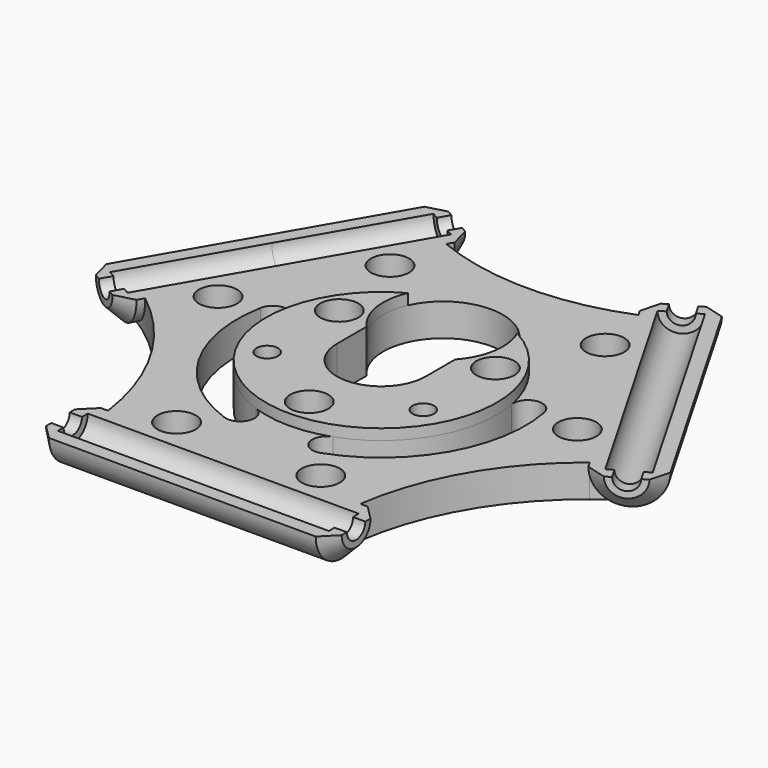
from build123d import *

# Parameters (mm, degrees)
F0_R            = 2.65
F0_R_2          = 1.5
F1_DEPTH        = 4.5
F2_R            = 1.6
F3_DEPTH        = 70.8788764306
F3_COPIES_COUNT = 3
F5_R            = 2.6
F6_DEPTH        = 18.8
F6_DEPTH_BACK   = 18.8
F6_COPIES_COUNT = 3
F8_T1_DEPTH     = 63.5
F8_T3_DEPTH     = 63.5
F8_T5_DEPTH     = 63.5
F8_T10_DEPTH    = 25.5
F8_S11_R        = 35.5
F8_T12_DEPTH    = 16
F8_T16_DEPTH    = 25.5
F8_S17_R        = 35.5
F8_T18_DEPTH    = 16
F8_T22_DEPTH    = 25.5
F8_S23_R        = 35.5
F8_T24_DEPTH    = 15
F8_T28_DEPTH    = 25.5
F8_S29_R        = 35.5
F8_T30_DEPTH    = 15
F8_T34_DEPTH    = 25.5
F8_S35_R        = 35.5
F8_T36_DEPTH    = 16
F8_T40_DEPTH    = 25.5
F8_S41_R        = 35.5
F8_T42_DEPTH    = 16
F9_SIZE         = 2
F10_R           = 1.5
F10_R_2         = 2.65
F11_DEPTH       = 1.5


# Not quite as in the source:
# - a fillet or chamfer that OpenCascade refuses, or shapes differently, is made with other operations: its cross-section is extruded or revolved along the edge and cut away or added
# - a pattern or mirror of a feature is missing from the dataset's text; its kind, count and spacing are read off the source's solid


with BuildPart() as f1:
    # F0 (on Top) → F1 (new body)
    with BuildSketch(Plane.XY):
        with BuildLine():
            Line((-40.1278764306, -0.5035207776), (-32.3336477965, -5.0035207776))
            Line((-32.3336477965, -5.0035207776), (-30.8336477965, -2.4054445662))
            ThreePointArc((-30.8336477965, -2.4054445662), (-21.9158664068, -12.6531313695), (-17.5, -25.5))
            Line((-17.5, -25.5), (-20.5, -25.5))
            Line((-20.5, -25.5), (-20.5, -34.5))
            Line((-20.5, -34.5), (20.5, -34.5))
            Line((20.5, -34.5), (20.5, -25.5))
            Line((20.5, -25.5), (17.5, -25.5))
            ThreePointArc((17.5, -25.5), (21.9158664068, -12.6531313695), (30.8336477965, -2.4054445662))
            Line((30.8336477965, -2.4054445662), (32.3336477965, -5.0035207776))
            Line((32.3336477965, -5.0035207776), (40.1278764306, -0.5035207776))
            Line((40.1278764306, -0.5035207776), (19.6278764306, 35.0035207776))
            Line((19.6278764306, 35.0035207776), (11.8336477965, 30.5035207776))
            Line((11.8336477965, 30.5035207776), (13.3336477965, 27.9054445662))
            ThreePointArc((13.3336477965, 27.9054445662), (0, 25.306262739), (-13.3336477965, 27.9054445662))
            Line((-13.3336477965, 27.9054445662), (-11.8336477965, 30.5035207776))
            Line((-11.8336477965, 30.5035207776), (-19.6278764306, 35.0035207776))
            Line((-19.6278764306, 35.0035207776), (-40.1278764306, -0.5035207776))
        make_face()
        with Locations((-10, -23)):
            Circle(F0_R, mode=Mode.SUBTRACT)
        with BuildLine():
            ThreePointArc((-19.6632649519, 3.6545877239), (-17.3314796843, 5.2554554467), (-15.7306119615, 2.9236701791))
            ThreePointArc((-15.7306119615, 2.9236701791), (-13.8564064606, -8), (-5.3333333333, -15.0849446653))
            ThreePointArc((-5.3333333333, -15.0849446653), (-4.1143819168, -17.6372294151), (-6.6666666667, -18.8561808316))
            ThreePointArc((-6.6666666667, -18.8561808316), (-17.3205080757, -10), (-19.6632649519, 3.6545877239))
        make_face(mode=Mode.SUBTRACT)
        with Locations((-10.8253175473, -6.25)):
            Circle(F0_R_2, mode=Mode.SUBTRACT)
        with Locations((10, -23)):
            Circle(F0_R, mode=Mode.SUBTRACT)
        with Locations((0, -12.5)):
            Circle(F0_R, mode=Mode.SUBTRACT)
        with BuildLine():
            ThreePointArc((5.3333333333, -15.0849446653), (13.8564064606, -8), (15.7306119615, 2.9236701791))
            ThreePointArc((15.7306119615, 2.9236701791), (17.3314796843, 5.2554554467), (19.6632649519, 3.6545877239))
            ThreePointArc((19.6632649519, 3.6545877239), (17.3205080757, -10), (6.6666666667, -18.8561808316))
            ThreePointArc((6.6666666667, -18.8561808316), (4.1143819168, -17.6372294151), (5.3333333333, -15.0849446653))
        make_face(mode=Mode.SUBTRACT)
        with Locations((10.8253175473, -6.25)):
            Circle(F0_R_2, mode=Mode.SUBTRACT)
        with Locations((-24.918584287, 2.8397459622)):
            Circle(F0_R, mode=Mode.SUBTRACT)
        with Locations((-10.8253175473, 6.25)):
            Circle(F0_R, mode=Mode.SUBTRACT)
        with BuildLine():
            ThreePointArc((6.15, 0), (0, -6.15), (-6.15, 0))
            Line((-6.15, 0), (-6.15, 5.1163952154))
            ThreePointArc((-6.15, 5.1163952154), (0, 18.990217961), (6.15, 5.1163952154))
            Line((6.15, 5.1163952154), (6.15, 0))
        make_face(mode=Mode.SUBTRACT)
        with Locations((-14.918584287, 20.1602540378)):
            Circle(F0_R, mode=Mode.SUBTRACT)
        with Locations((10.8253175473, 6.25)):
            Circle(F0_R, mode=Mode.SUBTRACT)
        with Locations((24.918584287, 2.8397459622)):
            Circle(F0_R, mode=Mode.SUBTRACT)
        with Locations((14.918584287, 20.1602540378)):
            Circle(F0_R, mode=Mode.SUBTRACT)
    extrude(amount=F1_DEPTH)

    # F2 (on face) → F3 (cut, through all)
    with BuildSketch(Plane(origin=(-10.25, -17.7535207776, 0), x_dir=(0.8660254038, -0.5, 0), z_dir=(-0.5, -0.8660254038, 0))):
        with Locations((-30, 4.5)):
            Circle(F2_R)
    f3 = extrude(amount=-F3_DEPTH, mode=Mode.SUBTRACT)

    # F3_copies: F3 ×3 about axis
    f3_copies_axis = Axis((0, 0, 0), (0, 0, 1))
    for i in range(1, F3_COPIES_COUNT):
        add(f3.rotate(f3_copies_axis, i * 360 / F3_COPIES_COUNT), mode=Mode.SUBTRACT)

    # F5 (on plane+point) → F6 (cut, two sides)
    with BuildSketch(Plane(origin=(0, 0, 0), x_dir=(0.8660254038, -0.5, 0), z_dir=(-0.5, -0.8660254038, 0))) as f6_sk:
        with Locations((-30, 4.5)):
            Circle(F5_R)
    f6 = extrude(amount=-F6_DEPTH, mode=Mode.SUBTRACT) + extrude(f6_sk.sketch, amount=F6_DEPTH_BACK, mode=Mode.SUBTRACT)

    # F6_copies: F6 ×3 about axis
    f6_copies_axis = Axis((0, 0, 0), (0, 0, 1))
    for i in range(1, F6_COPIES_COUNT):
        add(f6.rotate(f6_copies_axis, i * 360 / F6_COPIES_COUNT), mode=Mode.SUBTRACT)

    # F8: fillet of radius 4.5 on 9 edges, made by hand

    # F8_s2 → F8_t1 (cut)
    with BuildSketch(Plane(origin=(15.875, 27.4963065702, 0), x_dir=(0, 0, 1), z_dir=(-0.5, -0.8660254038, 0))):
        with BuildLine():
            ThreePointArc((4.5, 34.5), (1.3180194847, 33.1819805153), (0, 30))
            Line((0, 30), (0, 34.5))
            Line((0, 34.5), (4.5, 34.5))
        make_face()
    extrude(amount=F8_T1_DEPTH, mode=Mode.SUBTRACT)

    # F8_s4 → F8_t3 (cut)
    with BuildSketch(Plane.YZ.offset(-31.75)):
        with BuildLine():
            ThreePointArc((-30, 0), (-33.1819805153, 1.3180194847), (-34.5, 4.5))
            Line((-34.5, 4.5), (-34.5, 0))
            Line((-34.5, 0), (-30, 0))
        make_face()
    extrude(amount=F8_T3_DEPTH, mode=Mode.SUBTRACT)

    # F8_s6 → F8_t5 (cut)
    with BuildSketch(Plane(origin=(15.875, -27.4963065702, 0), x_dir=(0, 0, 1), z_dir=(-0.5, 0.8660254038, 0))):
        with BuildLine():
            ThreePointArc((0, 30), (1.3180194847, 33.1819805153), (4.5, 34.5))
            Line((4.5, 34.5), (0, 34.5))
            Line((0, 34.5), (0, 30))
        make_face()
    extrude(amount=F8_T5_DEPTH, mode=Mode.SUBTRACT)


with BuildPart() as f8_tool8:
    # F8_s9 → F8_t10 (new body)
    with BuildSketch(Plane(origin=(-15.875, -27.4963065702, 0), x_dir=(0, 0, 1), z_dir=(0.5, 0.8660254038, 0))):
        with BuildLine():
            ThreePointArc((0, -30), (1.3180194847, -26.8180194847), (4.5, -25.5))
            Line((4.5, -25.5), (0, -25.5))
            Line((0, -25.5), (0, -30))
        make_face()
    extrude(amount=F8_T10_DEPTH)

    # F8_s11 → F8_t12 (intersect, symmetric)
    with BuildSketch(Plane.XY.offset(2.3)):
        with Locations((-52.6597682412, -30.4031313695)):
            Circle(F8_S11_R)
    extrude(amount=F8_T12_DEPTH, both=True, mode=Mode.INTERSECT)


with BuildPart() as f1_1:
    add(f1.part)

    # F8_t7: cut F8_tool8
    add(f8_tool8.part, mode=Mode.SUBTRACT)


with BuildPart() as f8_tool14:
    # F8_s15 → F8_t16 (new body)
    with BuildSketch(Plane(origin=(3.125, 5.4126587737, 0), x_dir=(0, 0, 1), z_dir=(0.5, 0.8660254038, 0))):
        with BuildLine():
            ThreePointArc((0, -30), (1.3180194847, -26.8180194847), (4.5, -25.5))
            Line((4.5, -25.5), (0, -25.5))
            Line((0, -25.5), (0, -30))
        make_face()
    extrude(amount=F8_T16_DEPTH)

    # F8_s17 → F8_t18 (intersect, symmetric)
    with BuildSketch(Plane.XY.offset(2.2)):
        with Locations((0, 60.806262739)):
            Circle(F8_S17_R)
    extrude(amount=F8_T18_DEPTH, both=True, mode=Mode.INTERSECT)


with BuildPart() as f1_2:
    add(f1_1.part)

    # F8_t13: cut F8_tool14
    add(f8_tool14.part, mode=Mode.SUBTRACT)


with BuildPart() as f8_tool20:
    # F8_s21 → F8_t22 (new body)
    with BuildSketch(Plane.YZ.offset(-6.25)):
        with BuildLine():
            ThreePointArc((-30, 0), (-26.8180194847, 1.3180194847), (-25.5, 4.5))
            Line((-25.5, 4.5), (-25.5, 0))
            Line((-25.5, 0), (-30, 0))
        make_face()
    extrude(amount=-F8_T22_DEPTH)

    # F8_s23 → F8_t24 (intersect, symmetric)
    with BuildSketch(Plane.XY.offset(2.2)):
        with Locations((-52.6597682412, -30.4031313695)):
            Circle(F8_S23_R)
    extrude(amount=F8_T24_DEPTH, both=True, mode=Mode.INTERSECT)


with BuildPart() as f1_3:
    add(f1_2.part)

    # F8_t19: cut F8_tool20
    add(f8_tool20.part, mode=Mode.SUBTRACT)


with BuildPart() as f8_tool26:
    # F8_s27 → F8_t28 (new body)
    with BuildSketch(Plane.YZ.offset(31.75)):
        with BuildLine():
            ThreePointArc((-30, 0), (-26.8180194847, 1.3180194847), (-25.5, 4.5))
            Line((-25.5, 4.5), (-25.5, 0))
            Line((-25.5, 0), (-30, 0))
        make_face()
    extrude(amount=-F8_T28_DEPTH)

    # F8_s29 → F8_t30 (intersect, symmetric)
    with BuildSketch(Plane.XY.offset(2.2)):
        with Locations((52.6597682412, -30.4031313695)):
            Circle(F8_S29_R)
    extrude(amount=F8_T30_DEPTH, both=True, mode=Mode.INTERSECT)


with BuildPart() as f1_4:
    add(f1_3.part)

    # F8_t25: cut F8_tool26
    add(f8_tool26.part, mode=Mode.SUBTRACT)


with BuildPart() as f8_tool32:
    # F8_s33 → F8_t34 (new body)
    with BuildSketch(Plane(origin=(3.125, -5.4126587737, 0), x_dir=(0, 0, 1), z_dir=(0.5, -0.8660254038, 0))):
        with BuildLine():
            ThreePointArc((0, -30), (1.3180194847, -26.8180194847), (4.5, -25.5))
            Line((4.5, -25.5), (0, -25.5))
            Line((0, -25.5), (0, -30))
        make_face()
    extrude(amount=F8_T34_DEPTH)

    # F8_s35 → F8_t36 (intersect, symmetric)
    with BuildSketch(Plane.XY.offset(2.3)):
        with Locations((52.6597682412, -30.4031313695)):
            Circle(F8_S35_R)
    extrude(amount=F8_T36_DEPTH, both=True, mode=Mode.INTERSECT)


with BuildPart() as f1_5:
    add(f1_4.part)

    # F8_t31: cut F8_tool32
    add(f8_tool32.part, mode=Mode.SUBTRACT)


with BuildPart() as f8_tool38:
    # F8_s39 → F8_t40 (new body)
    with BuildSketch(Plane(origin=(-15.875, 27.4963065702, 0), x_dir=(0, 0, 1), z_dir=(0.5, -0.8660254038, 0))):
        with BuildLine():
            ThreePointArc((0, -30), (1.3180194847, -26.8180194847), (4.5, -25.5))
            Line((4.5, -25.5), (0, -25.5))
            Line((0, -25.5), (0, -30))
        make_face()
    extrude(amount=F8_T40_DEPTH)

    # F8_s41 → F8_t42 (intersect, symmetric)
    with BuildSketch(Plane.XY.offset(2.2)):
        with Locations((0, 60.806262739)):
            Circle(F8_S41_R)
    extrude(amount=F8_T42_DEPTH, both=True, mode=Mode.INTERSECT)


with BuildPart() as f1_6:
    add(f1_5.part)

    # F8_t37: cut F8_tool38
    add(f8_tool38.part, mode=Mode.SUBTRACT)

    # F9
    f9_edges = [f1_6.edges().sort_by_distance(p)[0] for p in [
        (-38.986438, -1.162531, 1.318019),
        (-20.5, -26.818019, 1.318019),
        (20.5, -33.181981, 1.318019),
        (33.475086, -4.344511, 1.318019),
        (-33.475086, -4.344511, 1.318019),
        (-18.486438, 34.344511, 1.318019),
        (-12.975086, 31.162531, 1.318019),
        (38.986438, -1.162531, 1.318019),
        (20.5, -26.818019, 1.318019),
        (-20.5, -33.181981, 1.318019),
        (12.975086, 31.162531, 1.318019),
        (18.486438, 34.344511, 1.318019),
    ]]
    chamfer(f9_edges, length=F9_SIZE)

    # F10 (on face) → F11 (join)
    with BuildSketch(Plane.XY.offset(4.5)):
        with BuildLine():
            ThreePointArc((-6.15, 5.1163952154), (-8.198308632, 9.3949436369), (-7.568803222, 14.0965675888))
            ThreePointArc((-7.568803222, 14.0965675888), (0, -16), (7.568803222, 14.0965675888))
            ThreePointArc((7.568803222, 14.0965675888), (8.198308632, 9.3949436369), (6.15, 5.1163952154))
            Line((6.15, 5.1163952154), (6.15, 0))
            ThreePointArc((6.15, 0), (0, -6.15), (-6.15, 0))
            Line((-6.15, 0), (-6.15, 5.1163952154))
        make_face()
        with Locations((-10.8253175473, -6.25)):
            Circle(F10_R, mode=Mode.SUBTRACT)
        with Locations((0, -12.5)):
            Circle(F10_R_2, mode=Mode.SUBTRACT)
        with Locations((10.8253175473, -6.25)):
            Circle(F10_R, mode=Mode.SUBTRACT)
        with Locations((-10.8253175473, 6.25)):
            Circle(F10_R_2, mode=Mode.SUBTRACT)
        with Locations((10.8253175473, 6.25)):
            Circle(F10_R_2, mode=Mode.SUBTRACT)
    extrude(amount=F11_DEPTH)


solid = f1_6.part
